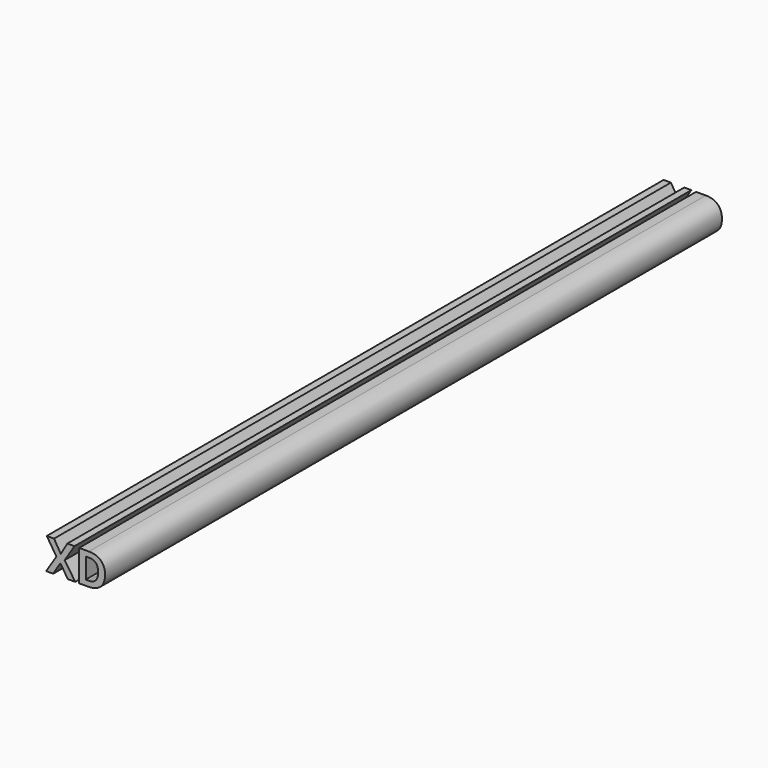
from build123d import *

# Parameters (mm, degrees)
F1_DEPTH     = 2514.6
F0_TEXT_SIZE = 142.5195278393
F2_DEPTH     = 2514.6


# Not quite as in the source:
# - Text() gives the source's letters only with a copy of the font that has no kerning and outlines rounded to 1/6400 em; it was checked with that copy


with BuildPart() as f1:
    # F0 (on Front) → F1 (new body)
    with BuildSketch(Plane.XZ):
        Polygon((-0.9130081582, -65.2561336756), (23.7161477465, -65.2561336756), (-10.6666883447, -13.9713723297), (21.2665933618, 36.4894479959), (-1.9596359408, 36.4894479959), (-23.471177174, -0.1202557178), (-45.3835545793, 36.4894479959), (-69.1887694637, 36.4894479959), (-37.5895179006, -12.7911324897), (-71.3488310575, -65.2561336756), (-48.2339451361, -65.2561336756), (-24.5846109853, -26.775861159), align=None)
    extrude(amount=F1_DEPTH)

    # F0 (on Front) → F2 (join)
    with BuildSketch(Plane.XZ):
        with Locations((-71.3488310575, -65.2561336756)):
            Text('XD', F0_TEXT_SIZE, font='Open Sans', font_style=FontStyle.BOLD, text_align=(TextAlign.LEFT, TextAlign.BOTTOM))
    extrude(amount=F2_DEPTH)


solid = f1.part
